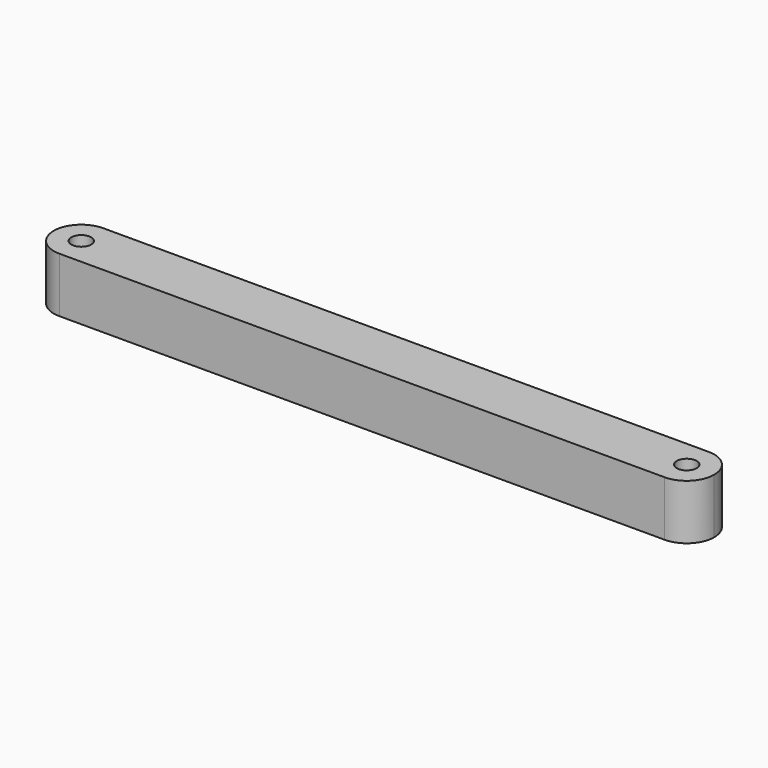
from build123d import *

# Parameters (mm, degrees)
F0_W     = 120
F0_H     = 10
F1_DEPTH = 5
F2_R     = 1.8
F3_DEPTH = 15
F4_R     = 4.99999
F5_R     = 1.8
F6_DEPTH = 11
F7_R     = 1.8
F8_DEPTH = 11


# Not quite as in the source:
# - a fillet or chamfer is up to 0.001 mm smaller than in the source, because OpenCascade refuses the exact size


with BuildPart() as f1:
    # F0 (on Top) → F1 (new body, symmetric)
    with BuildSketch(Plane.XY):
        with Locations((-46.6666666667, 0)):
            Rectangle(F0_W, F0_H)
    extrude(amount=F1_DEPTH, both=True)

    # F2 (on face) → F3 (cut)
    with BuildSketch(Plane.XY.offset(5)):
        with Locations((55.0279925401, -0.2576091507)):
            Circle(F2_R)
    extrude(amount=-F3_DEPTH, mode=Mode.SUBTRACT)

    # F4 (radius 5 in the source; OpenCascade refuses exactly that, so slightly less here)
    f4_edges = [f1.edges().sort_by_distance(p)[0] for p in [
        (13.333333, -5, 0),
        (13.333333, 5, 0),
        (-106.666667, -5, 0),
        (-106.666667, 5, 0),
    ]]
    fillet(f4_edges, radius=F4_R)

    # F5 (on face) → F6 (cut)
    with BuildSketch(Plane.XY.offset(5)):
        with Locations((-101.6666666667, 0)):
            Circle(F5_R)
    extrude(amount=-F6_DEPTH, mode=Mode.SUBTRACT)

    # F7 (on face) → F8 (cut)
    with BuildSketch(Plane.XY.offset(5)):
        with Locations((8.3333333333, 0)):
            Circle(F7_R)
    extrude(amount=-F8_DEPTH, mode=Mode.SUBTRACT)


solid = f1.part
